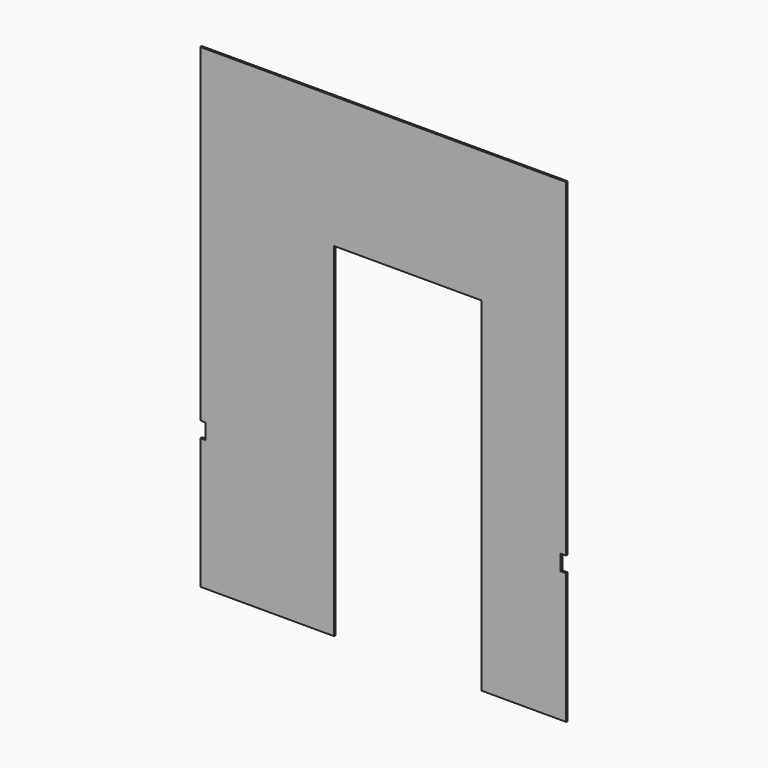
from build123d import *

# Parameters (mm, degrees)
F1_DEPTH = 12


# Not quite as in the source:
# - a feature names something its author has since deleted; it is built from what else it names


with BuildPart() as f1:
    # F0 (on Front) → F1 (new body)
    with BuildSketch(Plane.XZ):
        Polygon((1118, -557.5), (1118, 1452.5), (-1118, 1452.5), (-1118, -557.5), (-1085, -557.5), (-1085, -652.5), (-1118, -652.5), (-1118, -1452.5), (-300, -1452.5), (-300, 647.5), (600, 647.5), (600, -1452.5), (1118, -1452.5), (1118, -652.5), (1085, -652.5), (1085, -557.5), align=None)
    extrude(amount=F1_DEPTH)


solid = f1.part
